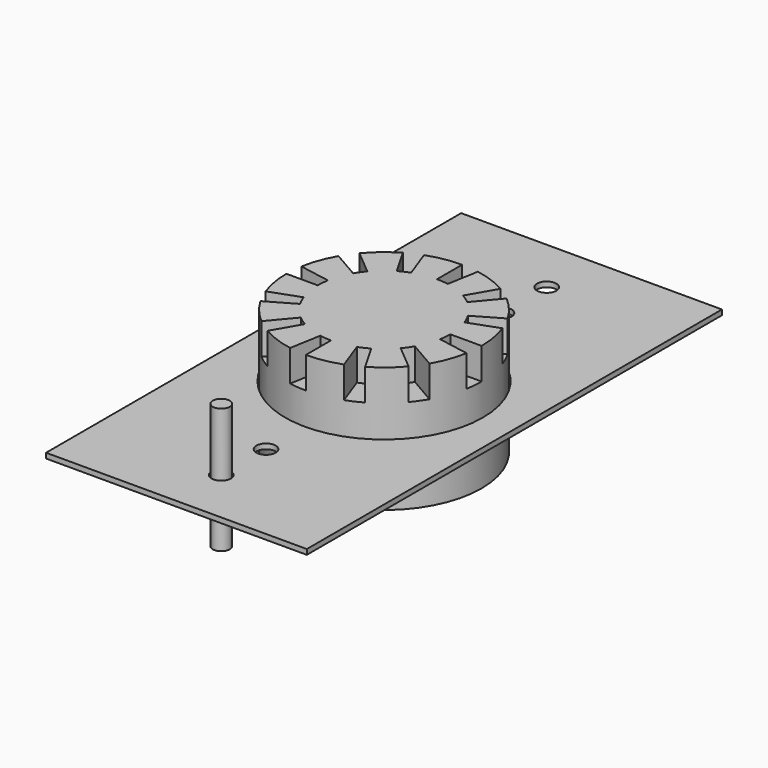
from build123d import *

# Parameters (mm, degrees)
F0_W            = 52.7812
F0_H            = 105.029
F0_R            = 1.9558
F0_R_2          = 20.0152
F1_DEPTH        = 1.0414
F2_R            = 19.7612
F3_DEPTH        = 12.7
F4_R            = 1.7018
F5_DEPTH        = 12.7
F7_DEPTH        = 6.35
F7_COPIES_COUNT = 12


# Not quite as in the source:
# - a pattern or mirror of a feature is missing from the dataset's text; its kind, count and spacing are read off the source's solid


with BuildPart() as f1:
    # F0 (on Top) → F1 (new body)
    with BuildSketch(Plane.XY):
        Rectangle(F0_W, F0_H)
        with Locations((0, -41.1734)):
            Circle(F0_R, mode=Mode.SUBTRACT)
        with Locations((0, -29.845)):
            Circle(F0_R, mode=Mode.SUBTRACT)
        Circle(F0_R_2, mode=Mode.SUBTRACT)
        with Locations((0, 29.845)):
            Circle(F0_R, mode=Mode.SUBTRACT)
        with Locations((0, 41.1734)):
            Circle(F0_R, mode=Mode.SUBTRACT)
    extrude(amount=F1_DEPTH)


with BuildPart() as f3:
    # F2 (on face) → F3 (new body, symmetric)
    with BuildSketch(Plane.XY.offset(1.0414)):
        Circle(F2_R)
    extrude(amount=F3_DEPTH, both=True)

    # F6 (on face) → F7 (cut)
    with BuildSketch(Plane.XY.offset(13.7414)):
        with BuildLine():
            ThreePointArc((0, 13.4112), (1.1688630971, 13.360166335), (2.3288304403, 13.2074537372))
            Line((2.3288304403, 13.2074537372), (3.4314963685, 19.4609829688))
            ThreePointArc((3.4314963685, 19.4609829688), (1.7223020636, 19.6860026679), (0, 19.7612))
            Line((0, 19.7612), (0, 13.4112))
        make_face()
    f7 = extrude(amount=-F7_DEPTH, mode=Mode.SUBTRACT)

    # F7_copies: F7 ×12 about axis
    f7_copies_axis = Axis((0, 0, 0), (0, 0, 1))
    for i in range(1, F7_COPIES_COUNT):
        add(f7.rotate(f7_copies_axis, i * 360 / F7_COPIES_COUNT), mode=Mode.SUBTRACT)


with BuildPart() as f5:
    # F4 (on face) → F5 (new body, symmetric)
    with BuildSketch(Plane.XY.offset(1.0414)):
        with Locations((0, -41.1734)):
            Circle(F4_R)
    extrude(amount=F5_DEPTH, both=True)


solid = Compound([f1.part, f3.part, f5.part])
